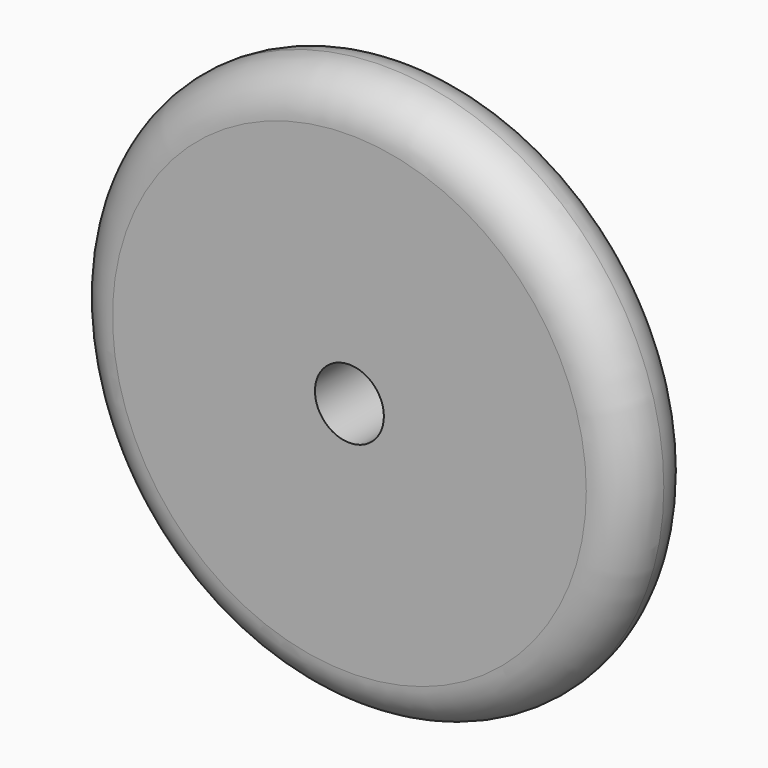
from build123d import *

# Parameters (mm, degrees)
F0_R     = 32.5
F0_R_2   = 4
F1_DEPTH = 10
F2_R     = 4.99999


# Not quite as in the source:
# - a fillet or chamfer is up to 0.001 mm smaller than in the source, because OpenCascade refuses the exact size


with BuildPart() as f1:
    # F0 (on Front) → F1 (new body)
    with BuildSketch(Plane.XZ):
        Circle(F0_R)
        Circle(F0_R_2, mode=Mode.SUBTRACT)
    extrude(amount=F1_DEPTH)

    # F2 (radius 5 in the source; OpenCascade refuses exactly that, so slightly less here)
    f2_edges = [f1.edges().sort_by_distance(p)[0] for p in [
        (-32.5, 0, 0),
        (-32.5, -10, 0),
    ]]
    fillet(f2_edges, radius=F2_R)


solid = f1.part
